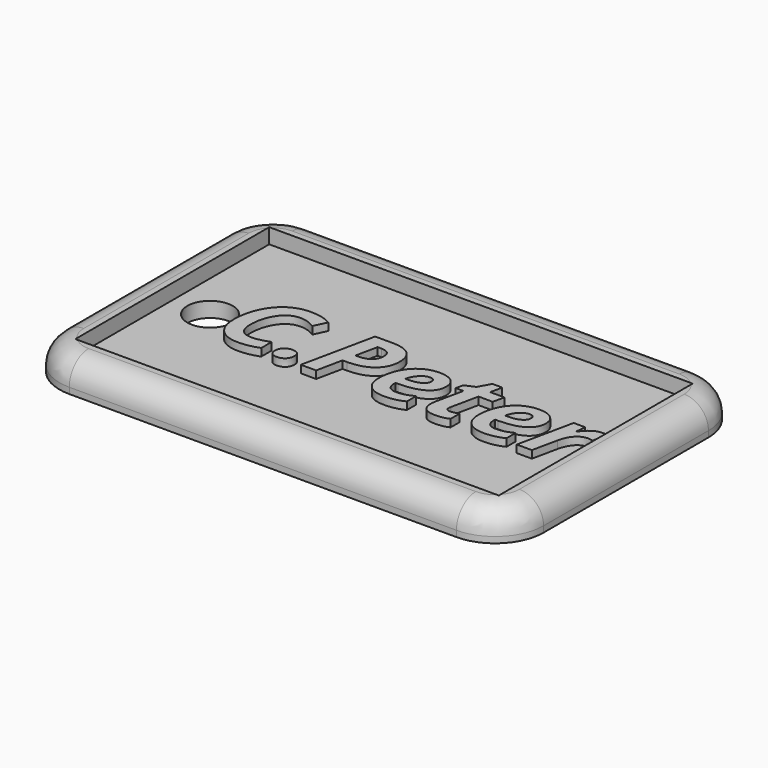
from build123d import *

# Parameters (mm, degrees)
F0_W         = 44.45
F0_H         = 25.4369186401
F0_R         = 2.38125
F1_DEPTH     = 1.5875
F0_W_2       = 50.8
F0_H_2       = 31.7869186401
F2_DEPTH     = 3.175
F3_R         = 5.08
F4_T1_DEPTH  = 40.64
F4_T3_DEPTH  = 21.6269186401
F4_T6_ANGLE  = 90
F4_T8_ANGLE  = 90
F4_T10_ANGLE = 90
F4_T12_ANGLE = 90
F5_TEXT_SIZE = 10.8099481314
F6_DEPTH     = 0.79375


# Not quite as in the source:
# - a fillet or chamfer that OpenCascade refuses, or shapes differently, is made with other operations: its cross-section is extruded or revolved along the edge and cut away or added
# - Text() gives the source's letters only with a copy of the font that has no kerning and outlines rounded to 1/6400 em; it was checked with that copy


with BuildPart() as f1:
    # F0 (on Top) → F1 (new body)
    with BuildSketch(Plane.XY):
        with Locations((25.4, 15.8934593201)):
            Rectangle(F0_W, F0_H)
        with Locations((7.14375, 15.8934593201)):
            Circle(F0_R, mode=Mode.SUBTRACT)
    extrude(amount=F1_DEPTH)

    # F0 (on Top) → F2 (join)
    with BuildSketch(Plane.XY):
        with Locations((25.4, 15.8934593201)):
            Rectangle(F0_W_2, F0_H_2)
        with Locations((25.4, 15.8934593201)):
            Rectangle(F0_W, F0_H, mode=Mode.SUBTRACT)
    extrude(amount=F2_DEPTH)

    # F3
    f3_edges = [f1.edges().sort_by_distance(p)[0] for p in [
        (50.8, 0, 1.5875),
        (50.8, 31.786919, 1.5875),
        (0, 0, 1.5875),
        (0, 31.786919, 1.5875),
    ]]
    fillet(f3_edges, radius=F3_R)

    # F4: fillet of radius 2.54 on 8 edges, made by hand

    # F4_s2 → F4_t1 (cut)
    with BuildSketch(Plane.YZ.offset(5.08)):
        with BuildLine():
            ThreePointArc((31.7869186401, 0.635), (31.0429698644, 2.4310512242), (29.2469186401, 3.175))
            Line((29.2469186401, 3.175), (31.7869186401, 3.175))
            Line((31.7869186401, 3.175), (31.7869186401, 0.635))
        make_face()
        with BuildLine():
            ThreePointArc((0, 0.635), (0.7439487758, 2.4310512242), (2.54, 3.175))
            Line((2.54, 3.175), (0, 3.175))
            Line((0, 3.175), (0, 0.635))
        make_face()
    extrude(amount=F4_T1_DEPTH, mode=Mode.SUBTRACT)

    # F4_s4 → F4_t3 (cut)
    with BuildSketch(Plane.XZ.offset(-26.7069186401)):
        with BuildLine():
            ThreePointArc((50.8, 0.635), (50.0560512242, 2.4310512242), (48.26, 3.175))
            Line((48.26, 3.175), (50.8, 3.175))
            Line((50.8, 3.175), (50.8, 0.635))
        make_face()
        with BuildLine():
            ThreePointArc((0, 0.635), (0.7439487758, 2.4310512242), (2.54, 3.175))
            Line((2.54, 3.175), (0, 3.175))
            Line((0, 3.175), (0, 0.635))
        make_face()
    extrude(amount=F4_T3_DEPTH, mode=Mode.SUBTRACT)

    # F4_s5 → F4_t6 (revolve, cut)
    with BuildSketch(Plane.XZ.offset(-26.7069186401)):
        with BuildLine():
            ThreePointArc((0, 0.635), (0.7439487758, 2.4310512242), (2.54, 3.175))
            Line((2.54, 3.175), (0, 3.175))
            Line((0, 3.175), (0, 0.635))
        make_face()
    revolve(axis=Axis((5.08, 26.7069186401, 3.175), (0, 0, -1)), revolution_arc=F4_T6_ANGLE, mode=Mode.SUBTRACT)

    # F4_s7 → F4_t8 (revolve, cut)
    with BuildSketch(Plane.XZ.offset(-5.08)):
        with BuildLine():
            ThreePointArc((0, 0.635), (0.7439487758, 2.4310512242), (2.54, 3.175))
            Line((2.54, 3.175), (0, 3.175))
            Line((0, 3.175), (0, 0.635))
        make_face()
    revolve(axis=Axis((5.08, 5.08, 3.175), (0, 0, 1)), revolution_arc=F4_T8_ANGLE, mode=Mode.SUBTRACT)

    # F4_s9 → F4_t10 (revolve, cut)
    with BuildSketch(Plane.XZ.offset(-26.7069186401)):
        with BuildLine():
            ThreePointArc((50.8, 0.635), (50.0560512242, 2.4310512242), (48.26, 3.175))
            Line((48.26, 3.175), (50.8, 3.175))
            Line((50.8, 3.175), (50.8, 0.635))
        make_face()
    revolve(axis=Axis((45.72, 26.7069186401, 3.175), (0, 0, 1)), revolution_arc=F4_T10_ANGLE, mode=Mode.SUBTRACT)

    # F4_s11 → F4_t12 (revolve, cut)
    with BuildSketch(Plane.YZ.offset(45.72)):
        with BuildLine():
            ThreePointArc((0, 0.635), (0.7439487758, 2.4310512242), (2.54, 3.175))
            Line((2.54, 3.175), (0, 3.175))
            Line((0, 3.175), (0, 0.635))
        make_face()
    revolve(axis=Axis((45.72, 5.08, 3.175), (0, 0, 1)), revolution_arc=F4_T12_ANGLE, mode=Mode.SUBTRACT)

    # F5 (on face) → F6 (join)
    with BuildSketch(Plane.XY.offset(1.5875)):
        with Locations((9.525, 12.3473987175)):
            Text('C.Peter', F5_TEXT_SIZE, font='Open Sans', font_style=FontStyle.BOLDITALIC, text_align=(TextAlign.LEFT, TextAlign.BOTTOM))
    extrude(amount=F6_DEPTH)


solid = f1.part
